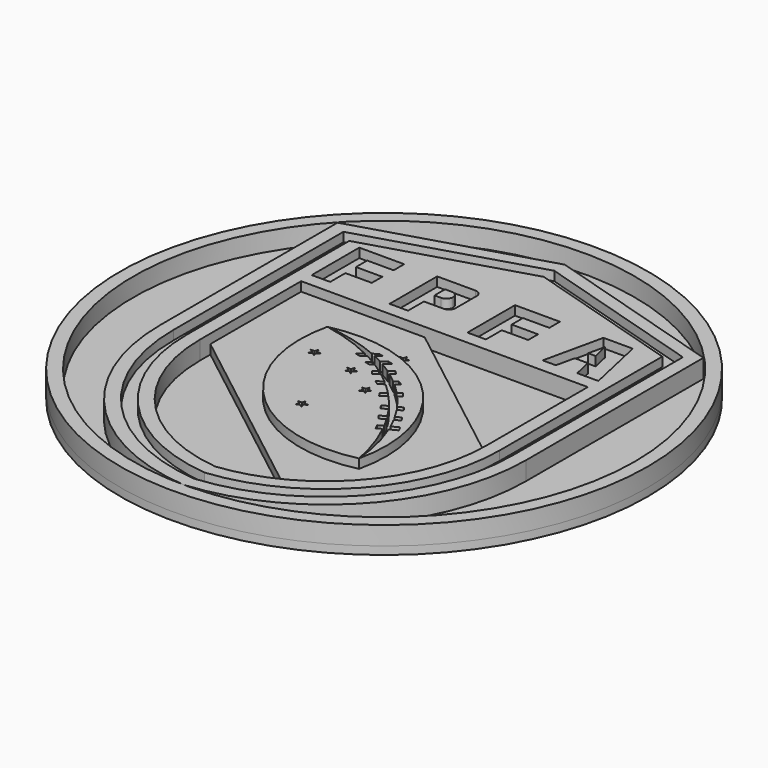
from build123d import *

# Parameters (mm, degrees)
F0_R     = 20
F1_DEPTH = 0.6
F2_R     = 20
F2_R_2   = 19
F3_DEPTH = 1.4
F4_W     = 1
F4_H     = 1
F5_DEPTH = 1.4
F6_DEPTH = 0.7
F7_DEPTH = 1.4
F8_R     = 0.49999
F9_R     = 0.49999


# Not quite as in the source:
# - a fillet or chamfer is up to 0.001 mm smaller than in the source, because OpenCascade refuses the exact size


with BuildPart() as f1:
    # F0 (on Top) → F1 (new body)
    with BuildSketch(Plane.XY):
        Circle(F0_R)
    extrude(amount=-F1_DEPTH)

    # F2 (on Top) → F3 (join)
    with BuildSketch(Plane.XY):
        Circle(F2_R)
        Circle(F2_R_2, mode=Mode.SUBTRACT)
    extrude(amount=F3_DEPTH)


with BuildPart() as f5:
    # F4 (on face) → F5 (new body)
    with BuildSketch(Plane.XY):
        with BuildLine():
            Line((13.86, 12.92), (0, 17.12))
            Line((0, 17.12), (-13.86, 12.92))
            Line((-13.86, 12.92), (-13.86, -3.88))
            ThreePointArc((-13.86, -3.88), (-9.8707167006, -14.1356569755), (0, -19))
            ThreePointArc((0, -19), (9.8707167006, -14.1356569755), (13.86, -3.88))
            Line((13.86, -3.88), (13.86, 12.92))
        make_face()
        with BuildLine():
            Line((-12.86, 12.223030303), (0, 16.12))
            Line((0, 16.12), (12.86, 12.223030303))
            Line((12.86, 12.223030303), (12.86, -3.88))
            ThreePointArc((12.86, -3.88), (9.1631609537, -13.4292669876), (0, -18))
            ThreePointArc((0, -18), (-9.1631609537, -13.4292669876), (-12.86, -3.88))
            Line((-12.86, -3.88), (-12.86, 12.223030303))
        make_face(mode=Mode.SUBTRACT)
        with BuildLine():
            Line((11.86, 11.5260606061), (0, 15.12))
            Line((0, 15.12), (-11.86, 11.5260606061))
            Line((-11.86, 11.5260606061), (-11.86, -3.88))
            ThreePointArc((-11.86, -3.88), (-8.4555353682, -12.7229915753), (0, -17))
            ThreePointArc((0, -17), (8.4555353682, -12.7229915753), (11.86, -3.88))
            Line((11.86, -3.88), (11.86, 11.5260606061))
        make_face()
        with BuildLine():
            Line((-10.86, -2.88), (-10.86, 5.72))
            Line((-10.86, 5.72), (-1.5, 5.72))
            Line((-1.5, 5.72), (10.86, 5.72))
            Line((10.86, 5.72), (10.86, -3.88))
            ThreePointArc((10.86, -3.88), (9.1005873506, -10.1895035062), (4.3301012314, -14.6781368788))
            ThreePointArc((4.3301012314, -14.6781368788), (2.2269405911, -15.5418049061), (0, -16))
            ThreePointArc((0, -16), (-7.747822298, -12.016860574), (-10.86, -3.88))
            Line((-10.86, -3.88), (-10.86, -2.88))
        make_face(mode=Mode.SUBTRACT)
        Polygon((-9.46, 6.72), (-10.86, 6.72), (-10.86, 11.2260606061), (-7.46, 11.2260606061), (-7.46, 10.2260606061), (-9.46, 10.2260606061), (-9.46, 9.1605855376), (-7.46, 9.1605855376), (-7.46, 8.1605855376), (-9.46, 8.1605855376), align=None, mode=Mode.SUBTRACT)
        Polygon((-3.56, 6.72), (-4.96, 6.72), (-4.96, 11.2260606061), (-1.56, 11.2260606061), (-1.56, 8.2260606061), (-3.56, 8.2260606061), align=None, mode=Mode.SUBTRACT)
        Polygon((0.94, 6.72), (0.94, 11.2260606061), (2.34, 11.2260606061), (4.34, 11.2260606061), (4.34, 10.2260606061), (2.34, 10.2260606061), (2.34, 9.1605855376), (4.34, 9.1605855376), (4.34, 8.2260606061), (2.34, 8.2260606061), (2.34, 6.72), align=None, mode=Mode.SUBTRACT)
        Polygon((7.64, 6.72), (6.64, 6.72), (7.64, 11.2260606061), (9.86, 11.2260606061), (10.86, 6.72), (9.26, 6.72), (8.9493073302, 8.12), (7.9506926698, 8.12), align=None, mode=Mode.SUBTRACT)
        with Locations((-3.06, 9.7260606061)):
            Rectangle(F4_W, F4_H)
        Polygon((8.45, 10.3699090909), (8.1726160054, 9.12), (8.7273839946, 9.12), align=None)
    extrude(amount=F5_DEPTH)

    # F8 (radius 0.5 in the source; OpenCascade refuses exactly that, so slightly less here)
    f8_edges = [f5.edges().sort_by_distance(p)[0] for p in [
        (-2.56, 9.226061, 0.7),
        (-2.56, 10.226061, 0.7),
        (-1.56, 11.226061, 0.7),
        (-1.56, 8.226061, 0.7),
    ]]
    fillet(f8_edges, radius=F8_R)


with BuildPart() as f6:
    # F4 (on face) → F6 (new body)
    with BuildSketch(Plane.XY):
        with BuildLine():
            Line((12.86, 12.223030303), (0, 16.12))
            Line((0, 16.12), (-12.86, 12.223030303))
            Line((-12.86, 12.223030303), (-12.86, -3.88))
            ThreePointArc((-12.86, -3.88), (-9.1631609537, -13.4292669876), (0, -18))
            ThreePointArc((0, -18), (9.1631609537, -13.4292669876), (12.86, -3.88))
            Line((12.86, -3.88), (12.86, 12.223030303))
        make_face()
        with BuildLine():
            Line((-11.86, 11.5260606061), (0, 15.12))
            Line((0, 15.12), (11.86, 11.5260606061))
            Line((11.86, 11.5260606061), (11.86, -3.88))
            ThreePointArc((11.86, -3.88), (8.4555353682, -12.7229915753), (0, -17))
            ThreePointArc((0, -17), (-8.4555353682, -12.7229915753), (-11.86, -3.88))
            Line((-11.86, -3.88), (-11.86, 11.5260606061))
        make_face(mode=Mode.SUBTRACT)
        with BuildLine():
            Line((-1.5, 5.72), (-10.86, 5.72))
            Line((-10.86, 5.72), (-10.86, -2.88))
            Line((-10.86, -2.88), (4.3301012314, -14.6781368788))
            ThreePointArc((4.3301012314, -14.6781368788), (9.1005873506, -10.1895035062), (10.86, -3.88))
            Line((10.86, -3.88), (-1.5, 5.72))
        make_face()
        with BuildLine():
            ThreePointArc((6, -9.88), (-3.3294104251, -7.2094104251), (-6, 2.12))
            ThreePointArc((-6, 2.12), (3.3294104251, -0.5505895749), (6, -9.88))
        make_face(mode=Mode.SUBTRACT)
        Polygon((-0.8796512219, 2.6644787905), (-1.1223563202, 2.8408143662), (-0.8223563202, 2.8408143662), (-0.7296512219, 3.1261313211), (-0.6369461236, 2.8408143662), (-0.3369461236, 2.8408143662), (-0.5796512219, 2.6644787905), (-0.4869461236, 2.3791618356), (-0.7296512219, 2.5554974113), (-0.9723563202, 2.3791618356), align=None, mode=Mode.SUBTRACT)
        Polygon((-4.96, 11.2260606061), (-4.96, 6.72), (-3.56, 6.72), (-3.56, 8.2260606061), (-1.56, 8.2260606061), (-1.56, 11.2260606061), align=None)
        with Locations((-3.06, 9.7260606061)):
            Rectangle(F4_W, F4_H, mode=Mode.SUBTRACT)
        Polygon((7.64, 11.2260606061), (6.64, 6.72), (7.64, 6.72), (7.9506926698, 8.12), (8.1726160054, 9.12), (8.45, 10.3699090909), (8.7273839946, 9.12), (8.9493073302, 8.12), (9.26, 6.72), (10.86, 6.72), (9.86, 11.2260606061), align=None)
        Polygon((-10.86, 11.2260606061), (-10.86, 6.72), (-9.46, 6.72), (-9.46, 8.1605855376), (-7.46, 8.1605855376), (-7.46, 9.1605855376), (-9.46, 9.1605855376), (-9.46, 10.2260606061), (-7.46, 10.2260606061), (-7.46, 11.2260606061), align=None)
        Polygon((2.34, 11.2260606061), (0.94, 11.2260606061), (0.94, 6.72), (2.34, 6.72), (2.34, 8.2260606061), (4.34, 8.2260606061), (4.34, 9.1605855376), (2.34, 9.1605855376), (2.34, 10.2260606061), (4.34, 10.2260606061), (4.34, 11.2260606061), align=None)
        with BuildLine():
            ThreePointArc((-1.7810191408, 1.0778315677), (-3.8466525454, 1.7764609322), (-6, 2.12))
            ThreePointArc((-6, 2.12), (-4.0135759202, 1.607338795), (-2.1156814582, 0.8284301053))
            Line((-2.1156814582, 0.8284301053), (-1.7810191408, 1.0778315677))
        make_face()
        with BuildLine():
            ThreePointArc((4.7329311685, -6.0456314878), (5.4960914693, -7.9199808108), (6, -9.88))
            ThreePointArc((6, -9.88), (5.6845091791, -7.8424772331), (5.0508523148, -5.8804597861))
            Line((5.0508523148, -5.8804597861), (4.7329311685, -6.0456314878))
        make_face()
        Polygon((8.1726160054, 9.12), (7.9506926698, 8.12), (8.9493073302, 8.12), (8.7273839946, 9.12), align=None)
        with BuildLine():
            ThreePointArc((2.3718156891, -2.5574328191), (2.7863940532, -3.0350765752), (3.1804686603, -3.5297724229))
            Line((3.1804686603, -3.5297724229), (3.6242615401, -3.3020057068))
            ThreePointArc((3.6242615401, -3.3020057068), (3.2195977495, -2.7639476832), (2.7876209555, -2.2475609389))
            Line((2.7876209555, -2.2475609389), (2.3718156891, -2.5574328191))
        make_face()
        with BuildLine():
            Line((1.7136965423, -1.164617013), (1.2909677714, -1.4796485184))
            ThreePointArc((1.2909677714, -1.4796485184), (1.701691498, -1.8636771599), (2.0977334355, -2.2628297132))
            Line((2.0977334355, -2.2628297132), (2.5172172214, -1.9502164782))
            ThreePointArc((2.5172172214, -1.9502164782), (2.1239494718, -1.5487304214), (1.7136965423, -1.164617013))
        make_face()
        with BuildLine():
            Line((0.6490416457, -0.3067067297), (0.2601613044, -0.63137253))
            ThreePointArc((0.2601613044, -0.63137253), (0.635842895, -0.9228815501), (1.0020957552, -1.2261520706))
            Line((1.0020957552, -1.2261520706), (1.4235077565, -0.9121018656))
            ThreePointArc((1.4235077565, -0.9121018656), (1.0419989313, -0.6020814401), (0.6490416457, -0.3067067297))
        make_face()
        with BuildLine():
            Line((-0.4656598313, 0.4149822015), (-0.8230655488, 0.1101466566))
            ThreePointArc((-0.8230655488, 0.1101466566), (-0.4442414233, -0.133481806), (-0.072902643, -0.3883740502))
            Line((-0.072902643, -0.3883740502), (0.3092255965, -0.0693453992))
            ThreePointArc((0.3092255965, -0.0693453992), (-0.0739602643, 0.1796290257), (-0.4656598313, 0.4149822015))
        make_face()
        with BuildLine():
            ThreePointArc((3.4193976106, -3.8518799308), (3.6800319471, -4.2250531272), (3.9292235304, -4.6059626264))
            Line((3.9292235304, -4.6059626264), (4.3239322068, -4.3960778547))
            ThreePointArc((4.3239322068, -4.3960778547), (4.0939609218, -4.0091954803), (3.850735243, -3.6305055904))
            Line((3.850735243, -3.6305055904), (3.4193976106, -3.8518799308))
        make_face()
        with BuildLine():
            ThreePointArc((4.1366160332, -4.9435129981), (4.3499336644, -5.3130623184), (4.5526536553, -5.6885296503))
            Line((4.5526536553, -5.6885296503), (4.8920268197, -5.5122128381))
            ThreePointArc((4.8920268197, -5.5122128381), (4.7097773777, -5.1241950969), (4.5148335191, -4.7423973513))
            Line((4.5148335191, -4.7423973513), (4.1366160332, -4.9435129981))
        make_face()
        with BuildLine():
            Line((-1.4699868837, 0.937727888), (-1.8186217191, 0.6779136416))
            ThreePointArc((-1.8186217191, 0.6779136416), (-1.4649878017, 0.4877107469), (-1.1165717348, 0.2881103136))
            Line((-1.1165717348, 0.2881103136), (-0.7689000691, 0.584643571))
            ThreePointArc((-0.7689000691, 0.584643571), (-1.1167778342, 0.7664786483), (-1.4699868837, 0.937727888))
        make_face()
        with BuildLine():
            ThreePointArc((4.8920268197, -5.5122128381), (4.972859661, -5.6957238234), (5.0508523148, -5.8804597861))
            Line((5.0508523148, -5.8804597861), (5.6022250712, -5.5940014066))
            Line((5.6022250712, -5.5940014066), (5.4178134377, -5.2390473962))
            Line((5.4178134377, -5.2390473962), (4.8920268197, -5.5122128381))
        make_face()
        with BuildLine():
            Line((1.9351058751, -2.8828834619), (2.3718156891, -2.5574328191))
            ThreePointArc((2.3718156891, -2.5574328191), (2.2357624674, -2.4092121745), (2.0977334355, -2.2628297132))
            Line((2.0977334355, -2.2628297132), (1.6960854764, -2.5621510983))
            Line((1.6960854764, -2.5621510983), (1.9351058751, -2.8828834619))
        make_face()
        with BuildLine():
            ThreePointArc((2.0977334355, -2.2628297132), (2.2357624674, -2.4092121745), (2.3718156891, -2.5574328191))
            Line((2.3718156891, -2.5574328191), (2.7876209555, -2.2475609389))
            ThreePointArc((2.7876209555, -2.2475609389), (2.6535682514, -2.0978436649), (2.5172172214, -1.9502164782))
            Line((2.5172172214, -1.9502164782), (2.0977334355, -2.2628297132))
        make_face()
        with BuildLine():
            Line((0.3092255965, -0.0693453992), (-0.072902643, -0.3883740502))
            ThreePointArc((-0.072902643, -0.3883740502), (0.0944642443, -0.5087289224), (0.2601613044, -0.63137253))
            Line((0.2601613044, -0.63137253), (0.6490416457, -0.3067067297))
            ThreePointArc((0.6490416457, -0.3067067297), (0.4800797171, -0.1866715953), (0.3092255965, -0.0693453992))
        make_face()
        with BuildLine():
            Line((3.7085615969, -5.1711292453), (4.1366160332, -4.9435129981))
            ThreePointArc((4.1366160332, -4.9435129981), (4.0340342292, -4.7740530906), (3.9292235304, -4.6059626264))
            Line((3.9292235304, -4.6059626264), (3.4695411982, -4.8503968817))
            Line((3.4695411982, -4.8503968817), (3.7085615969, -5.1711292453))
        make_face()
        with BuildLine():
            Line((1.4235077565, -0.9121018656), (1.0020957552, -1.2261520706))
            ThreePointArc((1.0020957552, -1.2261520706), (1.1473436767, -1.3519750782), (1.2909677714, -1.4796485184))
            Line((1.2909677714, -1.4796485184), (1.7136965423, -1.164617013))
            ThreePointArc((1.7136965423, -1.164617013), (1.5695361985, -1.037286036), (1.4235077565, -0.9121018656))
        make_face()
        with BuildLine():
            ThreePointArc((3.1804686603, -3.5297724229), (3.301009691, -3.6900276228), (3.4193976106, -3.8518799308))
            Line((3.4193976106, -3.8518799308), (3.850735243, -3.6305055904))
            ThreePointArc((3.850735243, -3.6305055904), (3.7387587742, -3.4653867183), (3.6242615401, -3.3020057068))
            Line((3.6242615401, -3.3020057068), (3.1804686603, -3.5297724229))
        make_face()
        with BuildLine():
            Line((2.9885739128, -4.0729905059), (3.4193976106, -3.8518799308))
            ThreePointArc((3.4193976106, -3.8518799308), (3.301009691, -3.6900276228), (3.1804686603, -3.5297724229))
            Line((3.1804686603, -3.5297724229), (2.7556631248, -3.7477943115))
            Line((2.7556631248, -3.7477943115), (2.9885739128, -4.0729905059))
        make_face()
        with BuildLine():
            ThreePointArc((1.2909677714, -1.4796485184), (1.1473436767, -1.3519750782), (1.0020957552, -1.2261520706))
            Line((1.0020957552, -1.2261520706), (0.5780526473, -1.5421630637))
            Line((0.5780526473, -1.5421630637), (0.9123552811, -1.761803108))
            Line((0.9123552811, -1.761803108), (1.2909677714, -1.4796485184))
        make_face()
        with BuildLine():
            ThreePointArc((0.2601613044, -0.63137253), (0.0944642443, -0.5087289224), (-0.072902643, -0.3883740502))
            Line((-0.072902643, -0.3883740502), (-0.3924984986, -0.6551960858))
            Line((-0.3924984986, -0.6551960858), (-0.1339669027, -0.9604196332))
            Line((-0.1339669027, -0.9604196332), (0.2601613044, -0.63137253))
        make_face()
        with BuildLine():
            ThreePointArc((4.3239322068, -4.3960778547), (4.4206997849, -4.5685116776), (4.5148335191, -4.7423973513))
            Line((4.5148335191, -4.7423973513), (4.9446694736, -4.5138337889))
            Line((4.9446694736, -4.5138337889), (4.705649075, -4.1931014254))
            Line((4.705649075, -4.1931014254), (4.3239322068, -4.3960778547))
        make_face()
        with BuildLine():
            Line((-0.3891848888, 0.9085071194), (-0.7689000691, 0.584643571))
            ThreePointArc((-0.7689000691, 0.584643571), (-0.6167130666, 0.5008260923), (-0.4656598313, 0.4149822015))
            Line((-0.4656598313, 0.4149822015), (-0.0012253545, 0.8111038354))
            Line((-0.0012253545, 0.8111038354), (-0.3891848888, 0.9085071194))
        make_face()
        with BuildLine():
            ThreePointArc((3.9292235304, -4.6059626264), (4.0340342292, -4.7740530906), (4.1366160332, -4.9435129981))
            Line((4.1366160332, -4.9435129981), (4.5148335191, -4.7423973513))
            ThreePointArc((4.5148335191, -4.7423973513), (4.4206997849, -4.5685116776), (4.3239322068, -4.3960778547))
            Line((4.3239322068, -4.3960778547), (3.9292235304, -4.6059626264))
        make_face()
        with BuildLine():
            Line((0.6821969357, 0.2420384006), (0.3092255965, -0.0693453992))
            ThreePointArc((0.3092255965, -0.0693453992), (0.4800797171, -0.1866715953), (0.6490416457, -0.3067067297))
            Line((0.6490416457, -0.3067067297), (0.9407285316, -0.0631851468))
            Line((0.9407285316, -0.0631851468), (0.6821969357, 0.2420384006))
        make_face()
        with BuildLine():
            Line((4.359886035, -6.2394421236), (4.7329311685, -6.0456314878))
            ThreePointArc((4.7329311685, -6.0456314878), (4.643982885, -5.8664795765), (4.5526536553, -5.6885296503))
            Line((4.5526536553, -5.6885296503), (4.1754744016, -5.8844881132))
            Line((4.1754744016, -5.8844881132), (4.359886035, -6.2394421236))
        make_face()
        with BuildLine():
            ThreePointArc((3.6242615401, -3.3020057068), (3.7387587742, -3.4653867183), (3.850735243, -3.6305055904))
            Line((3.850735243, -3.6305055904), (4.234112461, -3.4337458542))
            Line((4.234112461, -3.4337458542), (4.0012016731, -3.1085496597))
            Line((4.0012016731, -3.1085496597), (3.6242615401, -3.3020057068))
        make_face()
        with BuildLine():
            Line((-0.7689000691, 0.584643571), (-1.1165717348, 0.2881103136))
            ThreePointArc((-1.1165717348, 0.2881103136), (-0.9693095827, 0.1999680497), (-0.8230655488, 0.1101466566))
            Line((-0.8230655488, 0.1101466566), (-0.4656598313, 0.4149822015))
            ThreePointArc((-0.4656598313, 0.4149822015), (-0.6167130666, 0.5008260923), (-0.7689000691, 0.584643571))
        make_face()
        with BuildLine():
            ThreePointArc((-1.8186217191, 0.6779136416), (-1.9667338724, 0.7539962794), (-2.1156814582, 0.8284301053))
            Line((-2.1156814582, 0.8284301053), (-2.5679685297, 0.4913707735))
            Line((-2.5679685297, 0.4913707735), (-2.1760080285, 0.4115775064))
            Line((-2.1760080285, 0.4115775064), (-1.8186217191, 0.6779136416))
        make_face()
        with BuildLine():
            ThreePointArc((4.5526536553, -5.6885296503), (4.643982885, -5.8664795765), (4.7329311685, -6.0456314878))
            Line((4.7329311685, -6.0456314878), (5.0508523148, -5.8804597861))
            ThreePointArc((5.0508523148, -5.8804597861), (4.972859661, -5.6957238234), (4.8920268197, -5.5122128381))
            Line((4.8920268197, -5.5122128381), (4.5526536553, -5.6885296503))
        make_face()
        with BuildLine():
            ThreePointArc((2.5172172214, -1.9502164782), (2.6535682514, -2.0978436649), (2.7876209555, -2.2475609389))
            Line((2.7876209555, -2.2475609389), (3.0576691474, -2.0463120665))
            Line((3.0576691474, -2.0463120665), (2.8186487488, -1.725579703))
            Line((2.8186487488, -1.725579703), (2.5172172214, -1.9502164782))
        make_face()
        with BuildLine():
            Line((1.7006159197, -0.7055916684), (1.4235077565, -0.9121018656))
            ThreePointArc((1.4235077565, -0.9121018656), (1.5695361985, -1.037286036), (1.7136965423, -1.164617013))
            Line((1.7136965423, -1.164617013), (2.0349185535, -0.9252317127))
            Line((2.0349185535, -0.9252317127), (1.7006159197, -0.7055916684))
        make_face()
        with BuildLine():
            Line((-1.4454052573, 1.3279421688), (-1.7810191408, 1.0778315677))
            ThreePointArc((-1.7810191408, 1.0778315677), (-1.6250434381, 1.0087999894), (-1.4699868837, 0.937727888))
            Line((-1.4699868837, 0.937727888), (-1.0534447561, 1.2481489017))
            Line((-1.0534447561, 1.2481489017), (-1.4454052573, 1.3279421688))
        make_face()
        with BuildLine():
            Line((-1.7810191408, 1.0778315677), (-2.1156814582, 0.8284301053))
            ThreePointArc((-2.1156814582, 0.8284301053), (-1.9667338724, 0.7539962794), (-1.8186217191, 0.6779136416))
            Line((-1.8186217191, 0.6779136416), (-1.4699868837, 0.937727888))
            ThreePointArc((-1.4699868837, 0.937727888), (-1.6250434381, 1.0087999894), (-1.7810191408, 1.0778315677))
        make_face()
        with BuildLine():
            ThreePointArc((-0.8230655488, 0.1101466566), (-0.9693095827, 0.1999680497), (-1.1165717348, 0.2881103136))
            Line((-1.1165717348, 0.2881103136), (-1.4543678844, 0))
            Line((-1.4543678844, 0), (-1.0664083501, -0.0974032839))
            Line((-1.0664083501, -0.0974032839), (-0.8230655488, 0.1101466566))
        make_face()
    extrude(amount=F6_DEPTH)

    # F9 (radius 0.5 in the source; OpenCascade refuses exactly that, so slightly less here)
    f9_edges = [f6.edges().sort_by_distance(p)[0] for p in [
        (-2.56, 9.226061, 0.35),
        (-2.56, 10.226061, 0.35),
    ]]
    fillet(f9_edges, radius=F9_R)


with BuildPart() as f7:
    # F4 (on face) → F7 (new body)
    with BuildSketch(Plane.XY):
        with BuildLine():
            ThreePointArc((-2.1156814582, 0.8284301053), (-4.0135759202, 1.607338795), (-6, 2.12))
            ThreePointArc((-6, 2.12), (-3.3294104251, -7.2094104251), (6, -9.88))
            ThreePointArc((6, -9.88), (5.4960914693, -7.9199808108), (4.7329311685, -6.0456314878))
            Line((4.7329311685, -6.0456314878), (4.359886035, -6.2394421236))
            Line((4.359886035, -6.2394421236), (4.1754744016, -5.8844881132))
            Line((4.1754744016, -5.8844881132), (4.5526536553, -5.6885296503))
            ThreePointArc((4.5526536553, -5.6885296503), (4.3499336644, -5.3130623184), (4.1366160332, -4.9435129981))
            Line((4.1366160332, -4.9435129981), (3.7085615969, -5.1711292453))
            Line((3.7085615969, -5.1711292453), (3.4695411982, -4.8503968817))
            Line((3.4695411982, -4.8503968817), (3.9292235304, -4.6059626264))
            ThreePointArc((3.9292235304, -4.6059626264), (3.6800319471, -4.2250531272), (3.4193976106, -3.8518799308))
            Line((3.4193976106, -3.8518799308), (2.9885739128, -4.0729905059))
            Line((2.9885739128, -4.0729905059), (2.7556631248, -3.7477943115))
            Line((2.7556631248, -3.7477943115), (3.1804686603, -3.5297724229))
            ThreePointArc((3.1804686603, -3.5297724229), (2.7863940532, -3.0350765752), (2.3718156891, -2.5574328191))
            Line((2.3718156891, -2.5574328191), (1.9351058751, -2.8828834619))
            Line((1.9351058751, -2.8828834619), (1.6960854764, -2.5621510983))
            Line((1.6960854764, -2.5621510983), (2.0977334355, -2.2628297132))
            ThreePointArc((2.0977334355, -2.2628297132), (1.701691498, -1.8636771599), (1.2909677714, -1.4796485184))
            Line((1.2909677714, -1.4796485184), (0.9123552811, -1.761803108))
            Line((0.9123552811, -1.761803108), (0.5780526473, -1.5421630637))
            Line((0.5780526473, -1.5421630637), (1.0020957552, -1.2261520706))
            ThreePointArc((1.0020957552, -1.2261520706), (0.635842895, -0.9228815501), (0.2601613044, -0.63137253))
            Line((0.2601613044, -0.63137253), (-0.1339669027, -0.9604196332))
            Line((-0.1339669027, -0.9604196332), (-0.3924984986, -0.6551960858))
            Line((-0.3924984986, -0.6551960858), (-0.072902643, -0.3883740502))
            ThreePointArc((-0.072902643, -0.3883740502), (-0.4442414233, -0.133481806), (-0.8230655488, 0.1101466566))
            Line((-0.8230655488, 0.1101466566), (-1.0664083501, -0.0974032839))
            Line((-1.0664083501, -0.0974032839), (-1.4543678844, 0))
            Line((-1.4543678844, 0), (-1.1165717348, 0.2881103136))
            ThreePointArc((-1.1165717348, 0.2881103136), (-1.4649878017, 0.4877107469), (-1.8186217191, 0.6779136416))
            Line((-1.8186217191, 0.6779136416), (-2.1760080285, 0.4115775064))
            Line((-2.1760080285, 0.4115775064), (-2.5679685297, 0.4913707735))
            Line((-2.5679685297, 0.4913707735), (-2.1156814582, 0.8284301053))
        make_face()
        Polygon((-0.9355454553, -6.389078449), (-0.6355454553, -6.389078449), (-0.8782505536, -6.5654140247), (-0.7855454553, -6.8507309796), (-1.0282505536, -6.6743954039), (-1.270955652, -6.8507309796), (-1.1782505536, -6.5654140247), (-1.420955652, -6.389078449), (-1.120955652, -6.389078449), (-1.0282505536, -6.1037614942), align=None, mode=Mode.SUBTRACT)
        Polygon((-4.560217727, -1.0575196311), (-4.8029228253, -1.2338552068), (-4.710217727, -0.9485382519), (-4.9529228253, -0.7722026762), (-4.6529228253, -0.7722026762), (-4.560217727, -0.4868857213), (-4.4675126287, -0.7722026762), (-4.1675126287, -0.7722026762), (-4.410217727, -0.9485382519), (-4.3175126287, -1.2338552068), align=None, mode=Mode.SUBTRACT)
        Polygon((-1.4280958567, -1.5144857416), (-1.670800955, -1.6908213173), (-1.5780958567, -1.4055043624), (-1.820800955, -1.2291687867), (-1.520800955, -1.2291687867), (-1.4280958567, -0.9438518318), (-1.3353907584, -1.2291687867), (-1.0353907584, -1.2291687867), (-1.2780958567, -1.4055043624), (-1.1853907584, -1.6908213173), align=None, mode=Mode.SUBTRACT)
        Polygon((0.9208793904, -2.6571881003), (1.2208793904, -2.6571881003), (0.9781742921, -2.833523676), (1.0708793904, -3.1188406309), (0.8281742921, -2.9425050552), (0.5854691938, -3.1188406309), (0.6781742921, -2.833523676), (0.4354691938, -2.6571881003), (0.7354691938, -2.6571881003), (0.8281742921, -2.3718711454), align=None, mode=Mode.SUBTRACT)
        with BuildLine():
            ThreePointArc((6, -9.88), (3.3294104251, -0.5505895749), (-6, 2.12))
            ThreePointArc((-6, 2.12), (-3.8466525454, 1.7764609322), (-1.7810191408, 1.0778315677))
            Line((-1.7810191408, 1.0778315677), (-1.4454052573, 1.3279421688))
            Line((-1.4454052573, 1.3279421688), (-1.0534447561, 1.2481489017))
            Line((-1.0534447561, 1.2481489017), (-1.4699868837, 0.937727888))
            ThreePointArc((-1.4699868837, 0.937727888), (-1.1167778342, 0.7664786483), (-0.7689000691, 0.584643571))
            Line((-0.7689000691, 0.584643571), (-0.3891848888, 0.9085071194))
            Line((-0.3891848888, 0.9085071194), (-0.0012253545, 0.8111038354))
            Line((-0.0012253545, 0.8111038354), (-0.4656598313, 0.4149822015))
            ThreePointArc((-0.4656598313, 0.4149822015), (-0.0739602643, 0.1796290257), (0.3092255965, -0.0693453992))
            Line((0.3092255965, -0.0693453992), (0.6821969357, 0.2420384006))
            Line((0.6821969357, 0.2420384006), (0.9407285316, -0.0631851468))
            Line((0.9407285316, -0.0631851468), (0.6490416457, -0.3067067297))
            ThreePointArc((0.6490416457, -0.3067067297), (1.0419989313, -0.6020814401), (1.4235077565, -0.9121018656))
            Line((1.4235077565, -0.9121018656), (1.7006159197, -0.7055916684))
            Line((1.7006159197, -0.7055916684), (2.0349185535, -0.9252317127))
            Line((2.0349185535, -0.9252317127), (1.7136965423, -1.164617013))
            ThreePointArc((1.7136965423, -1.164617013), (2.1239494718, -1.5487304214), (2.5172172214, -1.9502164782))
            Line((2.5172172214, -1.9502164782), (2.8186487488, -1.725579703))
            Line((2.8186487488, -1.725579703), (3.0576691474, -2.0463120665))
            Line((3.0576691474, -2.0463120665), (2.7876209555, -2.2475609389))
            ThreePointArc((2.7876209555, -2.2475609389), (3.2195977495, -2.7639476832), (3.6242615401, -3.3020057068))
            Line((3.6242615401, -3.3020057068), (4.0012016731, -3.1085496597))
            Line((4.0012016731, -3.1085496597), (4.234112461, -3.4337458542))
            Line((4.234112461, -3.4337458542), (3.850735243, -3.6305055904))
            ThreePointArc((3.850735243, -3.6305055904), (4.0939609218, -4.0091954803), (4.3239322068, -4.3960778547))
            Line((4.3239322068, -4.3960778547), (4.705649075, -4.1931014254))
            Line((4.705649075, -4.1931014254), (4.9446694736, -4.5138337889))
            Line((4.9446694736, -4.5138337889), (4.5148335191, -4.7423973513))
            ThreePointArc((4.5148335191, -4.7423973513), (4.7097773777, -5.1241950969), (4.8920268197, -5.5122128381))
            Line((4.8920268197, -5.5122128381), (5.4178134377, -5.2390473962))
            Line((5.4178134377, -5.2390473962), (5.6022250712, -5.5940014066))
            Line((5.6022250712, -5.5940014066), (5.0508523148, -5.8804597861))
            ThreePointArc((5.0508523148, -5.8804597861), (5.6845091791, -7.8424772331), (6, -9.88))
        make_face()
    extrude(amount=F7_DEPTH)


solid = Compound([f1.part, f5.part, f6.part, f7.part])
